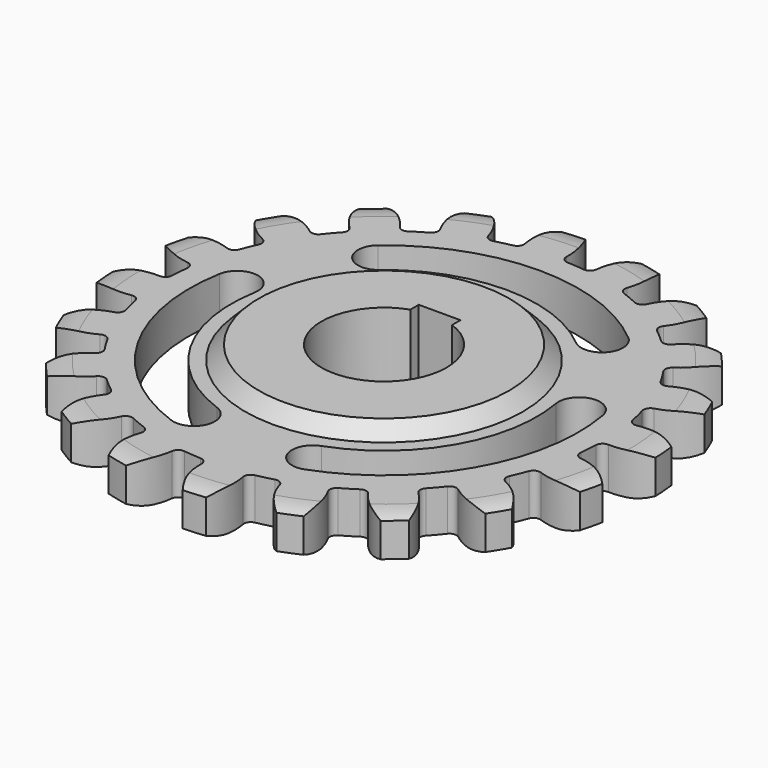
from build123d import *

# Parameters (mm, degrees)
F1_DEPTH = 3
F4_R     = 18
F5_DEPTH = 5
F6_SIZE  = 1.99999
F7_SIZE  = 1.99999


# Not quite as in the source:
# - a fillet or chamfer is up to 0.001 mm smaller than in the source, because OpenCascade refuses the exact size


with BuildPart() as f1:
    # F0 (on Top) → F1 (new body, symmetric)
    with BuildSketch(Plane.XY):
        with BuildLine():
            ThreePointArc((0.2738981657, 32.5091996366), (-0.108413774, 35.3828560798), (-1.4086644595, 37.9738813455))
            ThreePointArc((-1.4086644595, 37.9738813455), (-2.9813714286, 37.8828645222), (-4.5489545449, 37.7267413455))
            ThreePointArc((-4.5489545449, 37.7267413455), (-5.4278821585, 34.9642153234), (-5.3559596496, 32.0661313141))
            ThreePointArc((-5.3559596496, 32.0661313141), (-5.5077073558, 31.3183297867), (-6.1427227992, 30.8952578337))
            ThreePointArc((-6.1427227992, 30.8952578337), (-7.3534689607, 30.6296668974), (-8.5528286781, 30.3166475984))
            ThreePointArc((-8.5528286781, 30.3166475984), (-9.3107018811, 30.4053194594), (-9.785402526, 31.0027253419))
            ThreePointArc((-9.785402526, 31.0027253419), (-11.0370114644, 33.6175941412), (-13.0742941916, 35.6800060453))
            ThreePointArc((-13.0742941916, 35.6800060453), (-14.5419016576, 35.1074507218), (-15.9845170804, 34.4745589342))
            ThreePointArc((-15.9845170804, 34.4745589342), (-15.9667594264, 31.5756369901), (-15.0027998456, 28.8416205857))
            ThreePointArc((-15.0027998456, 28.8416205857), (-14.9160371102, 28.0835264501), (-15.3892362622, 27.4849305487))
            ThreePointArc((-15.3892362622, 27.4849305487), (-16.4586521758, 26.8581974182), (-17.5025827674, 26.1898758391))
            ThreePointArc((-17.5025827674, 26.1898758391), (-18.2507641276, 26.0400120911), (-18.8868398395, 26.461488282))
            ThreePointArc((-18.8868398395, 26.461488282), (-20.8852295733, 28.5616078606), (-23.4601209143, 29.8935231562))
            ThreePointArc((-23.4601209143, 29.8935231562), (-24.678969233, 28.8954750367), (-25.8554037134, 27.8477664961))
            ThreePointArc((-25.8554037134, 27.8477664961), (-24.9426990348, 25.0962153077), (-23.1810614622, 22.7938910831))
            ThreePointArc((-23.1810614622, 22.7938910831), (-22.864281226, 22.0997118752), (-23.1293440567, 21.3841867628))
            ThreePointArc((-23.1293440567, 21.3841867628), (-23.9527478417, 20.4576604437), (-24.7390621078, 19.4994565572))
            ThreePointArc((-24.7390621078, 19.4994565572), (-25.4043144208, 19.1257269079), (-26.1395016771, 19.330016381))
            ThreePointArc((-26.1395016771, 19.330016381), (-28.6890558956, 20.7098124021), (-31.5495075456, 21.1808539401))
            ThreePointArc((-31.5495075456, 21.1808539401), (-32.4002873514, 19.8550089285), (-33.1953832857, 18.4950406465))
            ThreePointArc((-33.1953832857, 18.4950406465), (-31.4770734756, 16.1602012154), (-29.0901992708, 14.5149367068))
            ThreePointArc((-29.0901992708, 14.5149367068), (-28.5744101906, 13.9526235241), (-28.6053905034, 13.1902097842))
            ThreePointArc((-28.6053905034, 13.1902097842), (-29.1021816603, 12.0545851281), (-29.5539096819, 10.9002946067))
            ThreePointArc((-29.5539096819, 10.9002946067), (-30.0711134162, 10.3392823182), (-30.833446966, 10.3063877965))
            ThreePointArc((-30.833446966, 10.3063877965), (-33.6845975384, 10.830796212), (-36.55060856, 10.3948551647))
            ThreePointArc((-36.55060856, 10.3948551647), (-36.9500395977, 8.8709962083), (-37.2859674562, 7.3318913559))
            ThreePointArc((-37.2859674562, 7.3318913559), (-34.9302526509, 5.6423140334), (-32.1517856915, 4.8151591942))
            ThreePointArc((-32.1517856915, 4.8151591942), (-31.4874767961, 4.4397551689), (-31.2813420221, 3.7050831703))
            ThreePointArc((-31.2813420221, 3.7050831703), (-31.4028911712, 2.4715230308), (-31.4758146622, 1.2341358733))
            ThreePointArc((-31.4758146622, 1.2341358733), (-31.7943423127, 0.5407567371), (-32.5091996366, 0.2738981657))
            ThreePointArc((-32.5091996366, 0.2738981657), (-35.3828560798, -0.108413774), (-37.9738813455, -1.4086644595))
            ThreePointArc((-37.9738813455, -1.4086644595), (-37.8828645222, -2.9813714286), (-37.7267413455, -4.5489545449))
            ThreePointArc((-37.7267413455, -4.5489545449), (-34.9642153234, -5.4278821585), (-32.0661313141, -5.3559596496))
            ThreePointArc((-32.0661313141, -5.3559596496), (-31.3183297867, -5.5077073558), (-30.8952578337, -6.1427227992))
            ThreePointArc((-30.8952578337, -6.1427227992), (-30.6296668974, -7.3534689607), (-30.3166475984, -8.5528286781))
            ThreePointArc((-30.3166475984, -8.5528286781), (-30.4053194594, -9.3107018811), (-31.0027253419, -9.785402526))
            ThreePointArc((-31.0027253419, -9.785402526), (-33.6175941412, -11.0370114644), (-35.6800060453, -13.0742941916))
            ThreePointArc((-35.6800060453, -13.0742941916), (-35.1074507218, -14.5419016576), (-34.4745589342, -15.9845170804))
            ThreePointArc((-34.4745589342, -15.9845170804), (-31.5756369901, -15.9667594264), (-28.8416205857, -15.0027998456))
            ThreePointArc((-28.8416205857, -15.0027998456), (-28.0835264501, -14.9160371102), (-27.4849305487, -15.3892362622))
            ThreePointArc((-27.4849305487, -15.3892362622), (-26.8581974182, -16.4586521758), (-26.1898758391, -17.5025827674))
            ThreePointArc((-26.1898758391, -17.5025827674), (-26.0400120911, -18.2507641276), (-26.461488282, -18.8868398395))
            ThreePointArc((-26.461488282, -18.8868398395), (-28.5616078606, -20.8852295733), (-29.8935231562, -23.4601209143))
            ThreePointArc((-29.8935231562, -23.4601209143), (-28.8954750367, -24.678969233), (-27.8477664961, -25.8554037134))
            ThreePointArc((-27.8477664961, -25.8554037134), (-25.0962153077, -24.9426990348), (-22.7938910831, -23.1810614622))
            ThreePointArc((-22.7938910831, -23.1810614622), (-22.0997118752, -22.864281226), (-21.3841867628, -23.1293440567))
            ThreePointArc((-21.3841867628, -23.1293440567), (-20.4576604437, -23.9527478417), (-19.4994565572, -24.7390621078))
            ThreePointArc((-19.4994565572, -24.7390621078), (-19.1257269079, -25.4043144208), (-19.330016381, -26.1395016771))
            ThreePointArc((-19.330016381, -26.1395016771), (-20.7098124021, -28.6890558956), (-21.1808539401, -31.5495075456))
            ThreePointArc((-21.1808539401, -31.5495075456), (-19.8550089285, -32.4002873514), (-18.4950406465, -33.1953832857))
            ThreePointArc((-18.4950406465, -33.1953832857), (-16.1602012154, -31.4770734756), (-14.5149367068, -29.0901992708))
            ThreePointArc((-14.5149367068, -29.0901992708), (-13.9526235241, -28.5744101906), (-13.1902097842, -28.6053905034))
            ThreePointArc((-13.1902097842, -28.6053905034), (-12.0545851281, -29.1021816603), (-10.9002946067, -29.5539096819))
            ThreePointArc((-10.9002946067, -29.5539096819), (-10.3392823182, -30.0711134162), (-10.3063877965, -30.833446966))
            ThreePointArc((-10.3063877965, -30.833446966), (-10.830796212, -33.6845975384), (-10.3948551647, -36.55060856))
            ThreePointArc((-10.3948551647, -36.55060856), (-8.8709962083, -36.9500395977), (-7.3318913559, -37.2859674562))
            ThreePointArc((-7.3318913559, -37.2859674562), (-5.6423140334, -34.9302526509), (-4.8151591942, -32.1517856915))
            ThreePointArc((-4.8151591942, -32.1517856915), (-4.4397551689, -31.4874767961), (-3.7050831703, -31.2813420221))
            ThreePointArc((-3.7050831703, -31.2813420221), (-2.4715230308, -31.4028911712), (-1.2341358733, -31.4758146622))
            ThreePointArc((-1.2341358733, -31.4758146622), (-0.5407567371, -31.7943423127), (-0.2738981657, -32.5091996366))
            ThreePointArc((-0.2738981657, -32.5091996366), (0.108413774, -35.3828560798), (1.4086644595, -37.9738813455))
            ThreePointArc((1.4086644595, -37.9738813455), (2.9813714286, -37.8828645222), (4.5489545449, -37.7267413455))
            ThreePointArc((4.5489545449, -37.7267413455), (5.4278821585, -34.9642153234), (5.3559596496, -32.0661313141))
            ThreePointArc((5.3559596496, -32.0661313141), (5.5077073558, -31.3183297867), (6.1427227992, -30.8952578337))
            ThreePointArc((6.1427227992, -30.8952578337), (7.3534689607, -30.6296668974), (8.5528286781, -30.3166475984))
            ThreePointArc((8.5528286781, -30.3166475984), (9.3107018811, -30.4053194594), (9.785402526, -31.0027253419))
            ThreePointArc((9.785402526, -31.0027253419), (11.0370114644, -33.6175941412), (13.0742941916, -35.6800060453))
            ThreePointArc((13.0742941916, -35.6800060453), (14.5419016576, -35.1074507218), (15.9845170804, -34.4745589342))
            ThreePointArc((15.9845170804, -34.4745589342), (15.9667594264, -31.5756369901), (15.0027998456, -28.8416205857))
            ThreePointArc((15.0027998456, -28.8416205857), (14.9160371102, -28.0835264501), (15.3892362622, -27.4849305487))
            ThreePointArc((15.3892362622, -27.4849305487), (16.4586521758, -26.8581974182), (17.5025827674, -26.1898758391))
            ThreePointArc((17.5025827674, -26.1898758391), (18.2507641276, -26.0400120911), (18.8868398395, -26.461488282))
            ThreePointArc((18.8868398395, -26.461488282), (20.8852295733, -28.5616078606), (23.4601209143, -29.8935231562))
            ThreePointArc((23.4601209143, -29.8935231562), (24.678969233, -28.8954750367), (25.8554037134, -27.8477664961))
            ThreePointArc((25.8554037134, -27.8477664961), (24.9426990348, -25.0962153077), (23.1810614622, -22.7938910831))
            ThreePointArc((23.1810614622, -22.7938910831), (22.864281226, -22.0997118752), (23.1293440567, -21.3841867628))
            ThreePointArc((23.1293440567, -21.3841867628), (23.9527478417, -20.4576604437), (24.7390621078, -19.4994565572))
            ThreePointArc((24.7390621078, -19.4994565572), (25.4043144208, -19.1257269079), (26.1395016771, -19.330016381))
            ThreePointArc((26.1395016771, -19.330016381), (28.6890558956, -20.7098124021), (31.5495075456, -21.1808539401))
            ThreePointArc((31.5495075456, -21.1808539401), (32.4002873514, -19.8550089285), (33.1953832857, -18.4950406465))
            ThreePointArc((33.1953832857, -18.4950406465), (31.4770734756, -16.1602012154), (29.0901992708, -14.5149367068))
            ThreePointArc((29.0901992708, -14.5149367068), (28.5744101906, -13.9526235241), (28.6053905034, -13.1902097842))
            ThreePointArc((28.6053905034, -13.1902097842), (29.1021816603, -12.0545851281), (29.5539096819, -10.9002946067))
            ThreePointArc((29.5539096819, -10.9002946067), (30.0711134162, -10.3392823182), (30.833446966, -10.3063877965))
            ThreePointArc((30.833446966, -10.3063877965), (33.6845975384, -10.830796212), (36.55060856, -10.3948551647))
            ThreePointArc((36.55060856, -10.3948551647), (36.9500395977, -8.8709962083), (37.2859674562, -7.3318913559))
            ThreePointArc((37.2859674562, -7.3318913559), (34.9302526509, -5.6423140334), (32.1517856915, -4.8151591942))
            ThreePointArc((32.1517856915, -4.8151591942), (31.4874767961, -4.4397551689), (31.2813420221, -3.7050831703))
            ThreePointArc((31.2813420221, -3.7050831703), (31.4028911712, -2.4715230308), (31.4758146622, -1.2341358733))
            ThreePointArc((31.4758146622, -1.2341358733), (31.7943423127, -0.5407567371), (32.5091996366, -0.2738981657))
            ThreePointArc((32.5091996366, -0.2738981657), (35.3828560798, 0.108413774), (37.9738813455, 1.4086644595))
            ThreePointArc((37.9738813455, 1.4086644595), (37.8828645222, 2.9813714286), (37.7267413455, 4.5489545449))
            ThreePointArc((37.7267413455, 4.5489545449), (34.9642153234, 5.4278821585), (32.0661313141, 5.3559596496))
            ThreePointArc((32.0661313141, 5.3559596496), (31.3183297867, 5.5077073558), (30.8952578337, 6.1427227992))
            ThreePointArc((30.8952578337, 6.1427227992), (30.6296668974, 7.3534689607), (30.3166475984, 8.5528286781))
            ThreePointArc((30.3166475984, 8.5528286781), (30.4053194594, 9.3107018811), (31.0027253419, 9.785402526))
            ThreePointArc((31.0027253419, 9.785402526), (33.6175941412, 11.0370114644), (35.6800060453, 13.0742941916))
            ThreePointArc((35.6800060453, 13.0742941916), (35.1074507218, 14.5419016576), (34.4745589342, 15.9845170804))
            ThreePointArc((34.4745589342, 15.9845170804), (31.5756369901, 15.9667594264), (28.8416205857, 15.0027998456))
            ThreePointArc((28.8416205857, 15.0027998456), (28.0835264501, 14.9160371102), (27.4849305487, 15.3892362622))
            ThreePointArc((27.4849305487, 15.3892362622), (26.8581974182, 16.4586521758), (26.1898758391, 17.5025827674))
            ThreePointArc((26.1898758391, 17.5025827674), (26.0400120911, 18.2507641276), (26.461488282, 18.8868398395))
            ThreePointArc((26.461488282, 18.8868398395), (28.5616078606, 20.8852295733), (29.8935231562, 23.4601209143))
            ThreePointArc((29.8935231562, 23.4601209143), (28.8954750367, 24.678969233), (27.8477664961, 25.8554037134))
            ThreePointArc((27.8477664961, 25.8554037134), (25.0962153077, 24.9426990348), (22.7938910831, 23.1810614622))
            ThreePointArc((22.7938910831, 23.1810614622), (22.0997118752, 22.864281226), (21.3841867628, 23.1293440567))
            ThreePointArc((21.3841867628, 23.1293440567), (20.4576604437, 23.9527478417), (19.4994565572, 24.7390621078))
            ThreePointArc((19.4994565572, 24.7390621078), (19.1257269079, 25.4043144208), (19.330016381, 26.1395016771))
            ThreePointArc((19.330016381, 26.1395016771), (20.7098124021, 28.6890558956), (21.1808539401, 31.5495075456))
            ThreePointArc((21.1808539401, 31.5495075456), (19.8550089285, 32.4002873514), (18.4950406465, 33.1953832857))
            ThreePointArc((18.4950406465, 33.1953832857), (16.1602012154, 31.4770734756), (14.5149367068, 29.0901992708))
            ThreePointArc((14.5149367068, 29.0901992708), (13.9526235241, 28.5744101906), (13.1902097842, 28.6053905034))
            ThreePointArc((13.1902097842, 28.6053905034), (12.0545851281, 29.1021816603), (10.9002946067, 29.5539096819))
            ThreePointArc((10.9002946067, 29.5539096819), (10.3392823182, 30.0711134162), (10.3063877965, 30.833446966))
            ThreePointArc((10.3063877965, 30.833446966), (10.830796212, 33.6845975384), (10.3948551647, 36.55060856))
            ThreePointArc((10.3948551647, 36.55060856), (8.8709962083, 36.9500395977), (7.3318913559, 37.2859674562))
            ThreePointArc((7.3318913559, 37.2859674562), (5.6423140334, 34.9302526509), (4.8151591942, 32.1517856915))
            ThreePointArc((4.8151591942, 32.1517856915), (4.4397551689, 31.4874767961), (3.7050831703, 31.2813420221))
            ThreePointArc((3.7050831703, 31.2813420221), (2.4715230308, 31.4028911712), (1.2341358733, 31.4758146622))
            ThreePointArc((1.2341358733, 31.4758146622), (0.5407567371, 31.7943423127), (0.2738981657, 32.5091996366))
        make_face()
        with BuildLine():
            ThreePointArc((-27.5746170843, 4.8621489747), (-24.0992492923, 7.2956277007), (-21.6657705663, 3.8202599087))
            ThreePointArc((-21.6657705663, 3.8202599087), (-19.0525588833, -11), (-7.5244431532, -20.6732376573))
            ThreePointArc((-7.5244431532, -20.6732376573), (-5.7314257208, -24.5183759496), (-9.5765640131, -26.311393382))
            ThreePointArc((-9.5765640131, -26.311393382), (-24.248711306, -14), (-27.5746170843, 4.8621489747))
        make_face(mode=Mode.SUBTRACT)
        with BuildLine():
            ThreePointArc((9.5765640131, -26.311393382), (5.7314257208, -24.5183759496), (7.5244431532, -20.6732376573))
            ThreePointArc((7.5244431532, -20.6732376573), (19.0525588833, -11), (21.6657705663, 3.8202599087))
            ThreePointArc((21.6657705663, 3.8202599087), (24.0992492923, 7.2956277007), (27.5746170843, 4.8621489747))
            ThreePointArc((27.5746170843, 4.8621489747), (24.248711306, -14), (9.5765640131, -26.311393382))
        make_face(mode=Mode.SUBTRACT)
        with BuildLine():
            ThreePointArc((3, 8.4852813742), (0, -9), (-3, 8.4852813742))
            Line((-3, 8.4852813742), (-3, 10))
            Line((-3, 10), (3, 10))
            Line((3, 10), (3, 8.4852813742))
        make_face(mode=Mode.SUBTRACT)
        with BuildLine():
            ThreePointArc((17.9980530712, 21.4492444073), (18.3678235715, 17.2227482489), (14.1413274131, 16.8529777486))
            ThreePointArc((14.1413274131, 16.8529777486), (0, 22), (-14.1413274131, 16.8529777486))
            ThreePointArc((-14.1413274131, 16.8529777486), (-18.3678235715, 17.2227482489), (-17.9980530712, 21.4492444073))
            ThreePointArc((-17.9980530712, 21.4492444073), (0, 28), (17.9980530712, 21.4492444073))
        make_face(mode=Mode.SUBTRACT)
    extrude(amount=F1_DEPTH, both=True)

    # F2 (on Right) → F3 (revolve, cut)
    with BuildSketch(Plane.YZ):
        with BuildLine():
            ThreePointArc((34.7261018343, 3), (36.3768398542, 2.871831403), (37.9738813455, 2.435))
            Line((37.9738813455, 2.435), (37.9738813455, -2.435))
            ThreePointArc((37.9738813455, -2.435), (36.3768398542, -2.871831403), (34.7261018343, -3))
            Line((34.7261018343, -3), (34.7261018343, -3.3218709417))
            Line((34.7261018343, -3.3218709417), (39.0829592943, -3.2214820385))
            Line((39.0829592943, -3.2214820385), (39.0829592943, 3.3296141773))
            Line((39.0829592943, 3.3296141773), (34.7261018343, 3.3296141773))
            Line((34.7261018343, 3.3296141773), (34.7261018343, 3))
        make_face()
    revolve(axis=Axis((0, 0, 0), (0, 0, 1)), mode=Mode.SUBTRACT)

    # F4 (on Top) → F5 (join, symmetric)
    with BuildSketch(Plane.XY):
        Circle(F4_R)
        with BuildLine():
            ThreePointArc((3, 8.4852813742), (0, -9), (-3, 8.4852813742))
            Line((-3, 8.4852813742), (-3, 10))
            Line((-3, 10), (3, 10))
            Line((3, 10), (3, 8.4852813742))
        make_face(mode=Mode.SUBTRACT)
    extrude(amount=F5_DEPTH, both=True)

    # F6 (size 2 in the source; OpenCascade refuses exactly that, so slightly less here)
    f6_edges = [f1.edges().sort_by_distance(p)[0] for p in [
        (-18, 0, 3),
    ]]
    chamfer(f6_edges, length=F6_SIZE)

    # F7 (size 2 in the source; OpenCascade refuses exactly that, so slightly less here)
    f7_edges = [f1.edges().sort_by_distance(p)[0] for p in [
        (-18, 0, -3),
    ]]
    chamfer(f7_edges, length=F7_SIZE)


solid = f1.part
